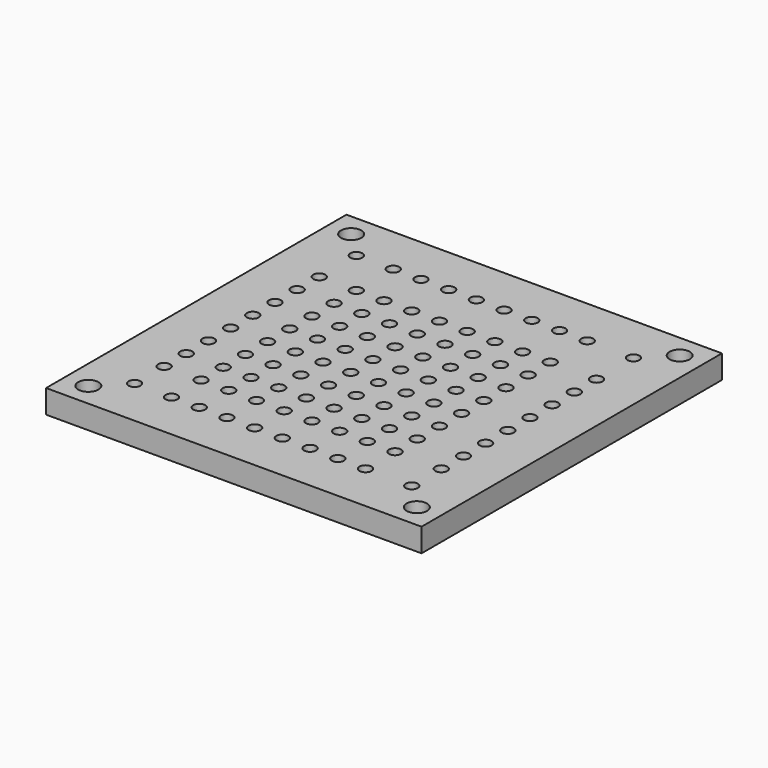
from build123d import *

# Parameters (mm, degrees)
F1_W     = 203.2
F1_H     = 203.2
F2_DEPTH = 12.7
F3_R     = 5.5
F3_R_2   = 3.25
F4_DEPTH = 6.35
F5_DEPTH = 12.701
F6_R     = 3.25
F7_DEPTH = 12.7
F8_DEPTH = 5


# Not quite as in the source:
# - a feature names something its author has since deleted; it is built from what else it names


with BuildPart() as f2:
    # F1 (on Top) → F2 (new body)
    with BuildSketch(Plane.XY):
        with Locations((101.6, 101.6)):
            Rectangle(F1_W, F1_H)
    extrude(amount=F2_DEPTH)

    # F3 (on face) → F4 (cut)
    with BuildSketch(Plane.XY.offset(12.7)):
        with Locations((12.7, 190.5)):
            Circle(F3_R)
        with Locations((12.7, 190.5)):
            Circle(F3_R_2, mode=Mode.SUBTRACT)
        with Locations((190.5, 190.5)):
            Circle(F3_R)
        with Locations((190.5, 190.5)):
            Circle(F3_R_2, mode=Mode.SUBTRACT)
        with Locations((190.5, 12.7)):
            Circle(F3_R)
        with Locations((190.5, 12.7)):
            Circle(F3_R_2, mode=Mode.SUBTRACT)
        with Locations((12.7, 12.7)):
            Circle(F3_R)
        with Locations((12.7, 12.7)):
            Circle(F3_R_2, mode=Mode.SUBTRACT)
        with Locations((12.7, 190.5)):
            Circle(F3_R_2)
        with Locations((190.5, 12.7)):
            Circle(F3_R_2)
        with Locations((190.5, 190.5)):
            Circle(F3_R_2)
        with Locations((12.7, 12.7)):
            Circle(F3_R_2)
    extrude(amount=-F4_DEPTH, mode=Mode.SUBTRACT)

    # F3 (on face) → F5 (cut, through all)
    with BuildSketch(Plane.XY.offset(12.7)):
        with Locations((12.7, 190.5)):
            Circle(F3_R_2)
        with Locations((190.5, 190.5)):
            Circle(F3_R_2)
        with Locations((190.5, 12.7)):
            Circle(F3_R_2)
        with Locations((12.7, 12.7)):
            Circle(F3_R_2)
    extrude(amount=-F5_DEPTH, mode=Mode.SUBTRACT)

    # F6 (on face) → F7 (cut, through all)
    with BuildSketch(Plane(origin=(0, 0, 0), x_dir=(1, 0, 0), z_dir=(0, 0, -1))):
        with Locations((26.6, -26.6)):
            Circle(F6_R)
        with Locations((46.6, -26.6)):
            Circle(F6_R)
        with Locations((61.6, -26.6)):
            Circle(F6_R)
        with Locations((76.6, -26.6)):
            Circle(F6_R)
        with Locations((91.6, -26.6)):
            Circle(F6_R)
        with Locations((106.6, -26.6)):
            Circle(F6_R)
        with Locations((121.6, -26.6)):
            Circle(F6_R)
        with Locations((136.6, -26.6)):
            Circle(F6_R)
        with Locations((151.6, -26.6)):
            Circle(F6_R)
        with Locations((176.6, -26.6)):
            Circle(F6_R)
        with Locations((176.6, -46.6)):
            Circle(F6_R)
        with Locations((151.6, -46.6)):
            Circle(F6_R)
        with Locations((136.6, -46.6)):
            Circle(F6_R)
        with Locations((121.6, -46.6)):
            Circle(F6_R)
        with Locations((106.6, -46.6)):
            Circle(F6_R)
        with Locations((91.6, -46.6)):
            Circle(F6_R)
        with Locations((76.6, -46.6)):
            Circle(F6_R)
        with Locations((61.6, -46.6)):
            Circle(F6_R)
        with Locations((46.6, -46.6)):
            Circle(F6_R)
        with Locations((26.6, -46.6)):
            Circle(F6_R)
        with Locations((26.6, -61.6)):
            Circle(F6_R)
        with Locations((46.6, -61.6)):
            Circle(F6_R)
        with Locations((61.6, -61.6)):
            Circle(F6_R)
        with Locations((76.6, -61.6)):
            Circle(F6_R)
        with Locations((91.6, -61.6)):
            Circle(F6_R)
        with Locations((106.6, -61.6)):
            Circle(F6_R)
        with Locations((121.6, -61.6)):
            Circle(F6_R)
        with Locations((136.6, -61.6)):
            Circle(F6_R)
        with Locations((151.6, -61.6)):
            Circle(F6_R)
        with Locations((176.6, -61.6)):
            Circle(F6_R)
        with Locations((176.6, -76.6)):
            Circle(F6_R)
        with Locations((151.6, -76.6)):
            Circle(F6_R)
        with Locations((136.6, -76.6)):
            Circle(F6_R)
        with Locations((121.6, -76.6)):
            Circle(F6_R)
        with Locations((106.6, -76.6)):
            Circle(F6_R)
        with Locations((91.6, -76.6)):
            Circle(F6_R)
        with Locations((76.6, -76.6)):
            Circle(F6_R)
        with Locations((61.6, -76.6)):
            Circle(F6_R)
        with Locations((46.6, -76.6)):
            Circle(F6_R)
        with Locations((26.6, -76.6)):
            Circle(F6_R)
        with Locations((26.6, -91.6)):
            Circle(F6_R)
        with Locations((46.6, -91.6)):
            Circle(F6_R)
        with Locations((61.6, -91.6)):
            Circle(F6_R)
        with Locations((76.6, -91.6)):
            Circle(F6_R)
        with Locations((91.6, -91.6)):
            Circle(F6_R)
        with Locations((106.6, -91.6)):
            Circle(F6_R)
        with Locations((121.6, -91.6)):
            Circle(F6_R)
        with Locations((136.6, -91.6)):
            Circle(F6_R)
        with Locations((151.6, -91.6)):
            Circle(F6_R)
        with Locations((176.6, -91.6)):
            Circle(F6_R)
        with Locations((176.6, -106.6)):
            Circle(F6_R)
        with Locations((151.6, -106.6)):
            Circle(F6_R)
        with Locations((136.6, -106.6)):
            Circle(F6_R)
        with Locations((121.6, -106.6)):
            Circle(F6_R)
        with Locations((106.6, -106.6)):
            Circle(F6_R)
        with Locations((91.6, -106.6)):
            Circle(F6_R)
        with Locations((76.6, -106.6)):
            Circle(F6_R)
        with Locations((61.6, -106.6)):
            Circle(F6_R)
        with Locations((46.6, -106.6)):
            Circle(F6_R)
        with Locations((26.6, -106.6)):
            Circle(F6_R)
        with Locations((26.6, -121.6)):
            Circle(F6_R)
        with Locations((46.6, -121.6)):
            Circle(F6_R)
        with Locations((61.6, -121.6)):
            Circle(F6_R)
        with Locations((76.6, -121.6)):
            Circle(F6_R)
        with Locations((91.6, -121.6)):
            Circle(F6_R)
        with Locations((106.6, -121.6)):
            Circle(F6_R)
        with Locations((121.6, -121.6)):
            Circle(F6_R)
        with Locations((136.6, -121.6)):
            Circle(F6_R)
        with Locations((151.6, -121.6)):
            Circle(F6_R)
        with Locations((176.6, -121.6)):
            Circle(F6_R)
        with Locations((176.6, -136.6)):
            Circle(F6_R)
        with Locations((151.6, -136.6)):
            Circle(F6_R)
        with Locations((136.6, -136.6)):
            Circle(F6_R)
        with Locations((121.6, -136.6)):
            Circle(F6_R)
        with Locations((106.6, -136.6)):
            Circle(F6_R)
        with Locations((91.6, -136.6)):
            Circle(F6_R)
        with Locations((76.6, -136.6)):
            Circle(F6_R)
        with Locations((61.6, -136.6)):
            Circle(F6_R)
        with Locations((46.6, -136.6)):
            Circle(F6_R)
        with Locations((26.6, -136.6)):
            Circle(F6_R)
        with Locations((26.6, -151.6)):
            Circle(F6_R)
        with Locations((46.6, -151.6)):
            Circle(F6_R)
        with Locations((61.6, -151.6)):
            Circle(F6_R)
        with Locations((76.6, -151.6)):
            Circle(F6_R)
        with Locations((91.6, -151.6)):
            Circle(F6_R)
        with Locations((106.6, -151.6)):
            Circle(F6_R)
        with Locations((121.6, -151.6)):
            Circle(F6_R)
        with Locations((136.6, -151.6)):
            Circle(F6_R)
        with Locations((151.6, -151.6)):
            Circle(F6_R)
        with Locations((176.6, -151.6)):
            Circle(F6_R)
        with Locations((176.6, -176.6)):
            Circle(F6_R)
        with Locations((151.6, -176.6)):
            Circle(F6_R)
        with Locations((136.6, -176.6)):
            Circle(F6_R)
        with Locations((121.6, -176.6)):
            Circle(F6_R)
        with Locations((106.6, -176.6)):
            Circle(F6_R)
        with Locations((91.6, -176.6)):
            Circle(F6_R)
        with Locations((76.6, -176.6)):
            Circle(F6_R)
        with Locations((61.6, -176.6)):
            Circle(F6_R)
        with Locations((46.6, -176.6)):
            Circle(F6_R)
        with Locations((26.6, -176.6)):
            Circle(F6_R)
    extrude(amount=-F7_DEPTH, mode=Mode.SUBTRACT)

    # F6 (on face) → F8 (cut)
    with BuildSketch(Plane(origin=(0, 0, 0), x_dir=(1, 0, 0), z_dir=(0, 0, -1))):
        Polygon((30.8457822208, -22.3542177792), (25.0459358482, -20.8001536274), (20.8001536274, -25.0459358482), (22.3542177792, -30.8457822208), (28.1540641518, -32.3998463726), (32.3998463726, -28.1540641518), align=None)
        with Locations((26.6, -26.6)):
            Circle(F6_R, mode=Mode.SUBTRACT)
        Polygon((50.8457822208, -22.3542177792), (45.0459358482, -20.8001536274), (40.8001536274, -25.0459358482), (42.3542177792, -30.8457822208), (48.1540641518, -32.3998463726), (52.3998463726, -28.1540641518), align=None)
        with Locations((46.6, -26.6)):
            Circle(F6_R, mode=Mode.SUBTRACT)
        Polygon((65.8457822208, -22.3542177792), (60.0459358482, -20.8001536274), (55.8001536274, -25.0459358482), (57.3542177792, -30.8457822208), (63.1540641518, -32.3998463726), (67.3998463726, -28.1540641518), align=None)
        with Locations((61.6, -26.6)):
            Circle(F6_R, mode=Mode.SUBTRACT)
        Polygon((80.8457822208, -22.3542177792), (75.0459358482, -20.8001536274), (70.8001536274, -25.0459358482), (72.3542177792, -30.8457822208), (78.1540641518, -32.3998463726), (82.3998463726, -28.1540641518), align=None)
        with Locations((76.6, -26.6)):
            Circle(F6_R, mode=Mode.SUBTRACT)
        Polygon((95.8457822208, -22.3542177792), (90.0459358482, -20.8001536274), (85.8001536274, -25.0459358482), (87.3542177792, -30.8457822208), (93.1540641518, -32.3998463726), (97.3998463726, -28.1540641518), align=None)
        with Locations((91.6, -26.6)):
            Circle(F6_R, mode=Mode.SUBTRACT)
        Polygon((110.8457822208, -22.3542177792), (105.0459358482, -20.8001536274), (100.8001536274, -25.0459358482), (102.3542177792, -30.8457822208), (108.1540641518, -32.3998463726), (112.3998463726, -28.1540641518), align=None)
        with Locations((106.6, -26.6)):
            Circle(F6_R, mode=Mode.SUBTRACT)
        Polygon((125.8457822208, -22.3542177792), (120.0459358482, -20.8001536274), (115.8001536274, -25.0459358482), (117.3542177792, -30.8457822208), (123.1540641518, -32.3998463726), (127.3998463726, -28.1540641518), align=None)
        with Locations((121.6, -26.6)):
            Circle(F6_R, mode=Mode.SUBTRACT)
        Polygon((140.8457822208, -22.3542177792), (135.0459358482, -20.8001536274), (130.8001536274, -25.0459358482), (132.3542177792, -30.8457822208), (138.1540641518, -32.3998463726), (142.3998463726, -28.1540641518), align=None)
        with Locations((136.6, -26.6)):
            Circle(F6_R, mode=Mode.SUBTRACT)
        Polygon((155.8457822208, -22.3542177792), (150.0459358482, -20.8001536274), (145.8001536274, -25.0459358482), (147.3542177792, -30.8457822208), (153.1540641518, -32.3998463726), (157.3998463726, -28.1540641518), align=None)
        with Locations((151.6, -26.6)):
            Circle(F6_R, mode=Mode.SUBTRACT)
        Polygon((180.8457822208, -22.3542177792), (175.0459358482, -20.8001536274), (170.8001536274, -25.0459358482), (172.3542177792, -30.8457822208), (178.1540641518, -32.3998463726), (182.3998463726, -28.1540641518), align=None)
        with Locations((176.6, -26.6)):
            Circle(F6_R, mode=Mode.SUBTRACT)
        Polygon((30.8457822208, -42.3542177792), (25.0459358482, -40.8001536274), (20.8001536274, -45.0459358482), (22.3542177792, -50.8457822208), (28.1540641518, -52.3998463726), (32.3998463726, -48.1540641518), align=None)
        with Locations((26.6, -46.6)):
            Circle(F6_R, mode=Mode.SUBTRACT)
        Polygon((50.8457822208, -42.3542177792), (45.0459358482, -40.8001536274), (40.8001536274, -45.0459358482), (42.3542177792, -50.8457822208), (48.1540641518, -52.3998463726), (52.3998463726, -48.1540641518), align=None)
        with Locations((46.6, -46.6)):
            Circle(F6_R, mode=Mode.SUBTRACT)
        Polygon((65.8457822208, -42.3542177792), (60.0459358482, -40.8001536274), (55.8001536274, -45.0459358482), (57.3542177792, -50.8457822208), (63.1540641518, -52.3998463726), (67.3998463726, -48.1540641518), align=None)
        with Locations((61.6, -46.6)):
            Circle(F6_R, mode=Mode.SUBTRACT)
        Polygon((80.8457822208, -42.3542177792), (75.0459358482, -40.8001536274), (70.8001536274, -45.0459358482), (72.3542177792, -50.8457822208), (78.1540641518, -52.3998463726), (82.3998463726, -48.1540641518), align=None)
        with Locations((76.6, -46.6)):
            Circle(F6_R, mode=Mode.SUBTRACT)
        Polygon((95.8457822208, -42.3542177792), (90.0459358482, -40.8001536274), (85.8001536274, -45.0459358482), (87.3542177792, -50.8457822208), (93.1540641518, -52.3998463726), (97.3998463726, -48.1540641518), align=None)
        with Locations((91.6, -46.6)):
            Circle(F6_R, mode=Mode.SUBTRACT)
        Polygon((110.8457822208, -42.3542177792), (105.0459358482, -40.8001536274), (100.8001536274, -45.0459358482), (102.3542177792, -50.8457822208), (108.1540641518, -52.3998463726), (112.3998463726, -48.1540641518), align=None)
        with Locations((106.6, -46.6)):
            Circle(F6_R, mode=Mode.SUBTRACT)
        Polygon((125.8457822208, -42.3542177792), (120.0459358482, -40.8001536274), (115.8001536274, -45.0459358482), (117.3542177792, -50.8457822208), (123.1540641518, -52.3998463726), (127.3998463726, -48.1540641518), align=None)
        with Locations((121.6, -46.6)):
            Circle(F6_R, mode=Mode.SUBTRACT)
        Polygon((140.8457822208, -42.3542177792), (135.0459358482, -40.8001536274), (130.8001536274, -45.0459358482), (132.3542177792, -50.8457822208), (138.1540641518, -52.3998463726), (142.3998463726, -48.1540641518), align=None)
        with Locations((136.6, -46.6)):
            Circle(F6_R, mode=Mode.SUBTRACT)
        Polygon((155.8457822208, -42.3542177792), (150.0459358482, -40.8001536274), (145.8001536274, -45.0459358482), (147.3542177792, -50.8457822208), (153.1540641518, -52.3998463726), (157.3998463726, -48.1540641518), align=None)
        with Locations((151.6, -46.6)):
            Circle(F6_R, mode=Mode.SUBTRACT)
        Polygon((180.8457822208, -42.3542177792), (175.0459358482, -40.8001536274), (170.8001536274, -45.0459358482), (172.3542177792, -50.8457822208), (178.1540641518, -52.3998463726), (182.3998463726, -48.1540641518), align=None)
        with Locations((176.6, -46.6)):
            Circle(F6_R, mode=Mode.SUBTRACT)
        Polygon((30.8457822208, -57.3542177792), (25.0459358482, -55.8001536274), (20.8001536274, -60.0459358482), (22.3542177792, -65.8457822208), (28.1540641518, -67.3998463726), (32.3998463726, -63.1540641518), align=None)
        with Locations((26.6, -61.6)):
            Circle(F6_R, mode=Mode.SUBTRACT)
        Polygon((50.8457822208, -57.3542177792), (45.0459358482, -55.8001536274), (40.8001536274, -60.0459358482), (42.3542177792, -65.8457822208), (48.1540641518, -67.3998463726), (52.3998463726, -63.1540641518), align=None)
        with Locations((46.6, -61.6)):
            Circle(F6_R, mode=Mode.SUBTRACT)
        Polygon((65.8457822208, -57.3542177792), (60.0459358482, -55.8001536274), (55.8001536274, -60.0459358482), (57.3542177792, -65.8457822208), (63.1540641518, -67.3998463726), (67.3998463726, -63.1540641518), align=None)
        with Locations((61.6, -61.6)):
            Circle(F6_R, mode=Mode.SUBTRACT)
        Polygon((80.8457822208, -57.3542177792), (75.0459358482, -55.8001536274), (70.8001536274, -60.0459358482), (72.3542177792, -65.8457822208), (78.1540641518, -67.3998463726), (82.3998463726, -63.1540641518), align=None)
        with Locations((76.6, -61.6)):
            Circle(F6_R, mode=Mode.SUBTRACT)
        Polygon((95.8457822208, -57.3542177792), (90.0459358482, -55.8001536274), (85.8001536274, -60.0459358482), (87.3542177792, -65.8457822208), (93.1540641518, -67.3998463726), (97.3998463726, -63.1540641518), align=None)
        with Locations((91.6, -61.6)):
            Circle(F6_R, mode=Mode.SUBTRACT)
        Polygon((110.8457822208, -57.3542177792), (105.0459358482, -55.8001536274), (100.8001536274, -60.0459358482), (102.3542177792, -65.8457822208), (108.1540641518, -67.3998463726), (112.3998463726, -63.1540641518), align=None)
        with Locations((106.6, -61.6)):
            Circle(F6_R, mode=Mode.SUBTRACT)
        Polygon((125.8457822208, -57.3542177792), (120.0459358482, -55.8001536274), (115.8001536274, -60.0459358482), (117.3542177792, -65.8457822208), (123.1540641518, -67.3998463726), (127.3998463726, -63.1540641518), align=None)
        with Locations((121.6, -61.6)):
            Circle(F6_R, mode=Mode.SUBTRACT)
        Polygon((140.8457822208, -57.3542177792), (135.0459358482, -55.8001536274), (130.8001536274, -60.0459358482), (132.3542177792, -65.8457822208), (138.1540641518, -67.3998463726), (142.3998463726, -63.1540641518), align=None)
        with Locations((136.6, -61.6)):
            Circle(F6_R, mode=Mode.SUBTRACT)
        Polygon((155.8457822208, -57.3542177792), (150.0459358482, -55.8001536274), (145.8001536274, -60.0459358482), (147.3542177792, -65.8457822208), (153.1540641518, -67.3998463726), (157.3998463726, -63.1540641518), align=None)
        with Locations((151.6, -61.6)):
            Circle(F6_R, mode=Mode.SUBTRACT)
        Polygon((180.8457822208, -57.3542177792), (175.0459358482, -55.8001536274), (170.8001536274, -60.0459358482), (172.3542177792, -65.8457822208), (178.1540641518, -67.3998463726), (182.3998463726, -63.1540641518), align=None)
        with Locations((176.6, -61.6)):
            Circle(F6_R, mode=Mode.SUBTRACT)
        Polygon((30.8457822208, -72.3542177792), (25.0459358482, -70.8001536274), (20.8001536274, -75.0459358482), (22.3542177792, -80.8457822208), (28.1540641518, -82.3998463726), (32.3998463726, -78.1540641518), align=None)
        with Locations((26.6, -76.6)):
            Circle(F6_R, mode=Mode.SUBTRACT)
        Polygon((50.8457822208, -72.3542177792), (45.0459358482, -70.8001536274), (40.8001536274, -75.0459358482), (42.3542177792, -80.8457822208), (48.1540641518, -82.3998463726), (52.3998463726, -78.1540641518), align=None)
        with Locations((46.6, -76.6)):
            Circle(F6_R, mode=Mode.SUBTRACT)
        Polygon((65.8457822208, -72.3542177792), (60.0459358482, -70.8001536274), (55.8001536274, -75.0459358482), (57.3542177792, -80.8457822208), (63.1540641518, -82.3998463726), (67.3998463726, -78.1540641518), align=None)
        with Locations((61.6, -76.6)):
            Circle(F6_R, mode=Mode.SUBTRACT)
        Polygon((80.8457822208, -72.3542177792), (75.0459358482, -70.8001536274), (70.8001536274, -75.0459358482), (72.3542177792, -80.8457822208), (78.1540641518, -82.3998463726), (82.3998463726, -78.1540641518), align=None)
        with Locations((76.6, -76.6)):
            Circle(F6_R, mode=Mode.SUBTRACT)
        Polygon((95.8457822208, -72.3542177792), (90.0459358482, -70.8001536274), (85.8001536274, -75.0459358482), (87.3542177792, -80.8457822208), (93.1540641518, -82.3998463726), (97.3998463726, -78.1540641518), align=None)
        with Locations((91.6, -76.6)):
            Circle(F6_R, mode=Mode.SUBTRACT)
        Polygon((110.8457822208, -72.3542177792), (105.0459358482, -70.8001536274), (100.8001536274, -75.0459358482), (102.3542177792, -80.8457822208), (108.1540641518, -82.3998463726), (112.3998463726, -78.1540641518), align=None)
        with Locations((106.6, -76.6)):
            Circle(F6_R, mode=Mode.SUBTRACT)
        Polygon((125.8457822208, -72.3542177792), (120.0459358482, -70.8001536274), (115.8001536274, -75.0459358482), (117.3542177792, -80.8457822208), (123.1540641518, -82.3998463726), (127.3998463726, -78.1540641518), align=None)
        with Locations((121.6, -76.6)):
            Circle(F6_R, mode=Mode.SUBTRACT)
        Polygon((140.8457822208, -72.3542177792), (135.0459358482, -70.8001536274), (130.8001536274, -75.0459358482), (132.3542177792, -80.8457822208), (138.1540641518, -82.3998463726), (142.3998463726, -78.1540641518), align=None)
        with Locations((136.6, -76.6)):
            Circle(F6_R, mode=Mode.SUBTRACT)
        Polygon((155.8457822208, -72.3542177792), (150.0459358482, -70.8001536274), (145.8001536274, -75.0459358482), (147.3542177792, -80.8457822208), (153.1540641518, -82.3998463726), (157.3998463726, -78.1540641518), align=None)
        with Locations((151.6, -76.6)):
            Circle(F6_R, mode=Mode.SUBTRACT)
        Polygon((180.8457822208, -72.3542177792), (175.0459358482, -70.8001536274), (170.8001536274, -75.0459358482), (172.3542177792, -80.8457822208), (178.1540641518, -82.3998463726), (182.3998463726, -78.1540641518), align=None)
        with Locations((176.6, -76.6)):
            Circle(F6_R, mode=Mode.SUBTRACT)
        Polygon((30.8457822208, -87.3542177792), (25.0459358482, -85.8001536274), (20.8001536274, -90.0459358482), (22.3542177792, -95.8457822208), (28.1540641518, -97.3998463726), (32.3998463726, -93.1540641518), align=None)
        with Locations((26.6, -91.6)):
            Circle(F6_R, mode=Mode.SUBTRACT)
        Polygon((50.8457822208, -87.3542177792), (45.0459358482, -85.8001536274), (40.8001536274, -90.0459358482), (42.3542177792, -95.8457822208), (48.1540641518, -97.3998463726), (52.3998463726, -93.1540641518), align=None)
        with Locations((46.6, -91.6)):
            Circle(F6_R, mode=Mode.SUBTRACT)
        Polygon((65.8457822208, -87.3542177792), (60.0459358482, -85.8001536274), (55.8001536274, -90.0459358482), (57.3542177792, -95.8457822208), (63.1540641518, -97.3998463726), (67.3998463726, -93.1540641518), align=None)
        with Locations((61.6, -91.6)):
            Circle(F6_R, mode=Mode.SUBTRACT)
        Polygon((80.8457822208, -87.3542177792), (75.0459358482, -85.8001536274), (70.8001536274, -90.0459358482), (72.3542177792, -95.8457822208), (78.1540641518, -97.3998463726), (82.3998463726, -93.1540641518), align=None)
        with Locations((76.6, -91.6)):
            Circle(F6_R, mode=Mode.SUBTRACT)
        Polygon((95.8457822208, -87.3542177792), (90.0459358482, -85.8001536274), (85.8001536274, -90.0459358482), (87.3542177792, -95.8457822208), (93.1540641518, -97.3998463726), (97.3998463726, -93.1540641518), align=None)
        with Locations((91.6, -91.6)):
            Circle(F6_R, mode=Mode.SUBTRACT)
        Polygon((110.8457822208, -87.3542177792), (105.0459358482, -85.8001536274), (100.8001536274, -90.0459358482), (102.3542177792, -95.8457822208), (108.1540641518, -97.3998463726), (112.3998463726, -93.1540641518), align=None)
        with Locations((106.6, -91.6)):
            Circle(F6_R, mode=Mode.SUBTRACT)
        Polygon((125.8457822208, -87.3542177792), (120.0459358482, -85.8001536274), (115.8001536274, -90.0459358482), (117.3542177792, -95.8457822208), (123.1540641518, -97.3998463726), (127.3998463726, -93.1540641518), align=None)
        with Locations((121.6, -91.6)):
            Circle(F6_R, mode=Mode.SUBTRACT)
        Polygon((140.8457822208, -87.3542177792), (135.0459358482, -85.8001536274), (130.8001536274, -90.0459358482), (132.3542177792, -95.8457822208), (138.1540641518, -97.3998463726), (142.3998463726, -93.1540641518), align=None)
        with Locations((136.6, -91.6)):
            Circle(F6_R, mode=Mode.SUBTRACT)
        Polygon((155.8457822208, -87.3542177792), (150.0459358482, -85.8001536274), (145.8001536274, -90.0459358482), (147.3542177792, -95.8457822208), (153.1540641518, -97.3998463726), (157.3998463726, -93.1540641518), align=None)
        with Locations((151.6, -91.6)):
            Circle(F6_R, mode=Mode.SUBTRACT)
        Polygon((180.8457822208, -87.3542177792), (175.0459358482, -85.8001536274), (170.8001536274, -90.0459358482), (172.3542177792, -95.8457822208), (178.1540641518, -97.3998463726), (182.3998463726, -93.1540641518), align=None)
        with Locations((176.6, -91.6)):
            Circle(F6_R, mode=Mode.SUBTRACT)
        Polygon((30.8457822208, -102.3542177792), (25.0459358482, -100.8001536274), (20.8001536274, -105.0459358482), (22.3542177792, -110.8457822208), (28.1540641518, -112.3998463726), (32.3998463726, -108.1540641518), align=None)
        with Locations((26.6, -106.6)):
            Circle(F6_R, mode=Mode.SUBTRACT)
        Polygon((50.8457822208, -102.3542177792), (45.0459358482, -100.8001536274), (40.8001536274, -105.0459358482), (42.3542177792, -110.8457822208), (48.1540641518, -112.3998463726), (52.3998463726, -108.1540641518), align=None)
        with Locations((46.6, -106.6)):
            Circle(F6_R, mode=Mode.SUBTRACT)
        Polygon((65.8457822208, -102.3542177792), (60.0459358482, -100.8001536274), (55.8001536274, -105.0459358482), (57.3542177792, -110.8457822208), (63.1540641518, -112.3998463726), (67.3998463726, -108.1540641518), align=None)
        with Locations((61.6, -106.6)):
            Circle(F6_R, mode=Mode.SUBTRACT)
        Polygon((80.8457822208, -102.3542177792), (75.0459358482, -100.8001536274), (70.8001536274, -105.0459358482), (72.3542177792, -110.8457822208), (78.1540641518, -112.3998463726), (82.3998463726, -108.1540641518), align=None)
        with Locations((76.6, -106.6)):
            Circle(F6_R, mode=Mode.SUBTRACT)
        Polygon((95.8457822208, -102.3542177792), (90.0459358482, -100.8001536274), (85.8001536274, -105.0459358482), (87.3542177792, -110.8457822208), (93.1540641518, -112.3998463726), (97.3998463726, -108.1540641518), align=None)
        with Locations((91.6, -106.6)):
            Circle(F6_R, mode=Mode.SUBTRACT)
        Polygon((110.8457822208, -102.3542177792), (105.0459358482, -100.8001536274), (100.8001536274, -105.0459358482), (102.3542177792, -110.8457822208), (108.1540641518, -112.3998463726), (112.3998463726, -108.1540641518), align=None)
        with Locations((106.6, -106.6)):
            Circle(F6_R, mode=Mode.SUBTRACT)
        Polygon((125.8457822208, -102.3542177792), (120.0459358482, -100.8001536274), (115.8001536274, -105.0459358482), (117.3542177792, -110.8457822208), (123.1540641518, -112.3998463726), (127.3998463726, -108.1540641518), align=None)
        with Locations((121.6, -106.6)):
            Circle(F6_R, mode=Mode.SUBTRACT)
        Polygon((140.8457822208, -102.3542177792), (135.0459358482, -100.8001536274), (130.8001536274, -105.0459358482), (132.3542177792, -110.8457822208), (138.1540641518, -112.3998463726), (142.3998463726, -108.1540641518), align=None)
        with Locations((136.6, -106.6)):
            Circle(F6_R, mode=Mode.SUBTRACT)
        Polygon((155.8457822208, -102.3542177792), (150.0459358482, -100.8001536274), (145.8001536274, -105.0459358482), (147.3542177792, -110.8457822208), (153.1540641518, -112.3998463726), (157.3998463726, -108.1540641518), align=None)
        with Locations((151.6, -106.6)):
            Circle(F6_R, mode=Mode.SUBTRACT)
        Polygon((180.8457822208, -102.3542177792), (175.0459358482, -100.8001536274), (170.8001536274, -105.0459358482), (172.3542177792, -110.8457822208), (178.1540641518, -112.3998463726), (182.3998463726, -108.1540641518), align=None)
        with Locations((176.6, -106.6)):
            Circle(F6_R, mode=Mode.SUBTRACT)
        Polygon((30.8457822208, -117.3542177792), (25.0459358482, -115.8001536274), (20.8001536274, -120.0459358482), (22.3542177792, -125.8457822208), (28.1540641518, -127.3998463726), (32.3998463726, -123.1540641518), align=None)
        with Locations((26.6, -121.6)):
            Circle(F6_R, mode=Mode.SUBTRACT)
        Polygon((50.8457822208, -117.3542177792), (45.0459358482, -115.8001536274), (40.8001536274, -120.0459358482), (42.3542177792, -125.8457822208), (48.1540641518, -127.3998463726), (52.3998463726, -123.1540641518), align=None)
        with Locations((46.6, -121.6)):
            Circle(F6_R, mode=Mode.SUBTRACT)
        Polygon((65.8457822208, -117.3542177792), (60.0459358482, -115.8001536274), (55.8001536274, -120.0459358482), (57.3542177792, -125.8457822208), (63.1540641518, -127.3998463726), (67.3998463726, -123.1540641518), align=None)
        with Locations((61.6, -121.6)):
            Circle(F6_R, mode=Mode.SUBTRACT)
        Polygon((80.8457822208, -117.3542177792), (75.0459358482, -115.8001536274), (70.8001536274, -120.0459358482), (72.3542177792, -125.8457822208), (78.1540641518, -127.3998463726), (82.3998463726, -123.1540641518), align=None)
        with Locations((76.6, -121.6)):
            Circle(F6_R, mode=Mode.SUBTRACT)
        Polygon((95.8457822208, -117.3542177792), (90.0459358482, -115.8001536274), (85.8001536274, -120.0459358482), (87.3542177792, -125.8457822208), (93.1540641518, -127.3998463726), (97.3998463726, -123.1540641518), align=None)
        with Locations((91.6, -121.6)):
            Circle(F6_R, mode=Mode.SUBTRACT)
        Polygon((110.8457822208, -117.3542177792), (105.0459358482, -115.8001536274), (100.8001536274, -120.0459358482), (102.3542177792, -125.8457822208), (108.1540641518, -127.3998463726), (112.3998463726, -123.1540641518), align=None)
        with Locations((106.6, -121.6)):
            Circle(F6_R, mode=Mode.SUBTRACT)
        Polygon((125.8457822208, -117.3542177792), (120.0459358482, -115.8001536274), (115.8001536274, -120.0459358482), (117.3542177792, -125.8457822208), (123.1540641518, -127.3998463726), (127.3998463726, -123.1540641518), align=None)
        with Locations((121.6, -121.6)):
            Circle(F6_R, mode=Mode.SUBTRACT)
        Polygon((140.8457822208, -117.3542177792), (135.0459358482, -115.8001536274), (130.8001536274, -120.0459358482), (132.3542177792, -125.8457822208), (138.1540641518, -127.3998463726), (142.3998463726, -123.1540641518), align=None)
        with Locations((136.6, -121.6)):
            Circle(F6_R, mode=Mode.SUBTRACT)
        Polygon((155.8457822208, -117.3542177792), (150.0459358482, -115.8001536274), (145.8001536274, -120.0459358482), (147.3542177792, -125.8457822208), (153.1540641518, -127.3998463726), (157.3998463726, -123.1540641518), align=None)
        with Locations((151.6, -121.6)):
            Circle(F6_R, mode=Mode.SUBTRACT)
        Polygon((180.8457822208, -117.3542177792), (175.0459358482, -115.8001536274), (170.8001536274, -120.0459358482), (172.3542177792, -125.8457822208), (178.1540641518, -127.3998463726), (182.3998463726, -123.1540641518), align=None)
        with Locations((176.6, -121.6)):
            Circle(F6_R, mode=Mode.SUBTRACT)
        Polygon((30.8457822208, -132.3542177792), (25.0459358482, -130.8001536274), (20.8001536274, -135.0459358482), (22.3542177792, -140.8457822208), (28.1540641518, -142.3998463726), (32.3998463726, -138.1540641518), align=None)
        with Locations((26.6, -136.6)):
            Circle(F6_R, mode=Mode.SUBTRACT)
        Polygon((50.8457822208, -132.3542177792), (45.0459358482, -130.8001536274), (40.8001536274, -135.0459358482), (42.3542177792, -140.8457822208), (48.1540641518, -142.3998463726), (52.3998463726, -138.1540641518), align=None)
        with Locations((46.6, -136.6)):
            Circle(F6_R, mode=Mode.SUBTRACT)
        Polygon((65.8457822208, -132.3542177792), (60.0459358482, -130.8001536274), (55.8001536274, -135.0459358482), (57.3542177792, -140.8457822208), (63.1540641518, -142.3998463726), (67.3998463726, -138.1540641518), align=None)
        with Locations((61.6, -136.6)):
            Circle(F6_R, mode=Mode.SUBTRACT)
        Polygon((80.8457822208, -132.3542177792), (75.0459358482, -130.8001536274), (70.8001536274, -135.0459358482), (72.3542177792, -140.8457822208), (78.1540641518, -142.3998463726), (82.3998463726, -138.1540641518), align=None)
        with Locations((76.6, -136.6)):
            Circle(F6_R, mode=Mode.SUBTRACT)
        Polygon((95.8457822208, -132.3542177792), (90.0459358482, -130.8001536274), (85.8001536274, -135.0459358482), (87.3542177792, -140.8457822208), (93.1540641518, -142.3998463726), (97.3998463726, -138.1540641518), align=None)
        with Locations((91.6, -136.6)):
            Circle(F6_R, mode=Mode.SUBTRACT)
        Polygon((110.8457822208, -132.3542177792), (105.0459358482, -130.8001536274), (100.8001536274, -135.0459358482), (102.3542177792, -140.8457822208), (108.1540641518, -142.3998463726), (112.3998463726, -138.1540641518), align=None)
        with Locations((106.6, -136.6)):
            Circle(F6_R, mode=Mode.SUBTRACT)
        Polygon((125.8457822208, -132.3542177792), (120.0459358482, -130.8001536274), (115.8001536274, -135.0459358482), (117.3542177792, -140.8457822208), (123.1540641518, -142.3998463726), (127.3998463726, -138.1540641518), align=None)
        with Locations((121.6, -136.6)):
            Circle(F6_R, mode=Mode.SUBTRACT)
        Polygon((140.8457822208, -132.3542177792), (135.0459358482, -130.8001536274), (130.8001536274, -135.0459358482), (132.3542177792, -140.8457822208), (138.1540641518, -142.3998463726), (142.3998463726, -138.1540641518), align=None)
        with Locations((136.6, -136.6)):
            Circle(F6_R, mode=Mode.SUBTRACT)
        Polygon((155.8457822208, -132.3542177792), (150.0459358482, -130.8001536274), (145.8001536274, -135.0459358482), (147.3542177792, -140.8457822208), (153.1540641518, -142.3998463726), (157.3998463726, -138.1540641518), align=None)
        with Locations((151.6, -136.6)):
            Circle(F6_R, mode=Mode.SUBTRACT)
        Polygon((180.8457822208, -132.3542177792), (175.0459358482, -130.8001536274), (170.8001536274, -135.0459358482), (172.3542177792, -140.8457822208), (178.1540641518, -142.3998463726), (182.3998463726, -138.1540641518), align=None)
        with Locations((176.6, -136.6)):
            Circle(F6_R, mode=Mode.SUBTRACT)
        Polygon((30.8457822208, -147.3542177792), (25.0459358482, -145.8001536274), (20.8001536274, -150.0459358482), (22.3542177792, -155.8457822208), (28.1540641518, -157.3998463726), (32.3998463726, -153.1540641518), align=None)
        with Locations((26.6, -151.6)):
            Circle(F6_R, mode=Mode.SUBTRACT)
        Polygon((50.8457822208, -147.3542177792), (45.0459358482, -145.8001536274), (40.8001536274, -150.0459358482), (42.3542177792, -155.8457822208), (48.1540641518, -157.3998463726), (52.3998463726, -153.1540641518), align=None)
        with Locations((46.6, -151.6)):
            Circle(F6_R, mode=Mode.SUBTRACT)
        Polygon((65.8457822208, -147.3542177792), (60.0459358482, -145.8001536274), (55.8001536274, -150.0459358482), (57.3542177792, -155.8457822208), (63.1540641518, -157.3998463726), (67.3998463726, -153.1540641518), align=None)
        with Locations((61.6, -151.6)):
            Circle(F6_R, mode=Mode.SUBTRACT)
        Polygon((80.8457822208, -147.3542177792), (75.0459358482, -145.8001536274), (70.8001536274, -150.0459358482), (72.3542177792, -155.8457822208), (78.1540641518, -157.3998463726), (82.3998463726, -153.1540641518), align=None)
        with Locations((76.6, -151.6)):
            Circle(F6_R, mode=Mode.SUBTRACT)
        Polygon((95.8457822208, -147.3542177792), (90.0459358482, -145.8001536274), (85.8001536274, -150.0459358482), (87.3542177792, -155.8457822208), (93.1540641518, -157.3998463726), (97.3998463726, -153.1540641518), align=None)
        with Locations((91.6, -151.6)):
            Circle(F6_R, mode=Mode.SUBTRACT)
        Polygon((110.8457822208, -147.3542177792), (105.0459358482, -145.8001536274), (100.8001536274, -150.0459358482), (102.3542177792, -155.8457822208), (108.1540641518, -157.3998463726), (112.3998463726, -153.1540641518), align=None)
        with Locations((106.6, -151.6)):
            Circle(F6_R, mode=Mode.SUBTRACT)
        Polygon((125.8457822208, -147.3542177792), (120.0459358482, -145.8001536274), (115.8001536274, -150.0459358482), (117.3542177792, -155.8457822208), (123.1540641518, -157.3998463726), (127.3998463726, -153.1540641518), align=None)
        with Locations((121.6, -151.6)):
            Circle(F6_R, mode=Mode.SUBTRACT)
        Polygon((140.8457822208, -147.3542177792), (135.0459358482, -145.8001536274), (130.8001536274, -150.0459358482), (132.3542177792, -155.8457822208), (138.1540641518, -157.3998463726), (142.3998463726, -153.1540641518), align=None)
        with Locations((136.6, -151.6)):
            Circle(F6_R, mode=Mode.SUBTRACT)
        Polygon((155.8457822208, -147.3542177792), (150.0459358482, -145.8001536274), (145.8001536274, -150.0459358482), (147.3542177792, -155.8457822208), (153.1540641518, -157.3998463726), (157.3998463726, -153.1540641518), align=None)
        with Locations((151.6, -151.6)):
            Circle(F6_R, mode=Mode.SUBTRACT)
        Polygon((180.8457822208, -147.3542177792), (175.0459358482, -145.8001536274), (170.8001536274, -150.0459358482), (172.3542177792, -155.8457822208), (178.1540641518, -157.3998463726), (182.3998463726, -153.1540641518), align=None)
        with Locations((176.6, -151.6)):
            Circle(F6_R, mode=Mode.SUBTRACT)
        Polygon((30.8457822208, -172.3542177792), (25.0459358482, -170.8001536274), (20.8001536274, -175.0459358482), (22.3542177792, -180.8457822208), (28.1540641518, -182.3998463726), (32.3998463726, -178.1540641518), align=None)
        with Locations((26.6, -176.6)):
            Circle(F6_R, mode=Mode.SUBTRACT)
        Polygon((50.8457822208, -172.3542177792), (45.0459358482, -170.8001536274), (40.8001536274, -175.0459358482), (42.3542177792, -180.8457822208), (48.1540641518, -182.3998463726), (52.3998463726, -178.1540641518), align=None)
        with Locations((46.6, -176.6)):
            Circle(F6_R, mode=Mode.SUBTRACT)
        Polygon((65.8457822208, -172.3542177792), (60.0459358482, -170.8001536274), (55.8001536274, -175.0459358482), (57.3542177792, -180.8457822208), (63.1540641518, -182.3998463726), (67.3998463726, -178.1540641518), align=None)
        with Locations((61.6, -176.6)):
            Circle(F6_R, mode=Mode.SUBTRACT)
        Polygon((80.8457822208, -172.3542177792), (75.0459358482, -170.8001536274), (70.8001536274, -175.0459358482), (72.3542177792, -180.8457822208), (78.1540641518, -182.3998463726), (82.3998463726, -178.1540641518), align=None)
        with Locations((76.6, -176.6)):
            Circle(F6_R, mode=Mode.SUBTRACT)
        Polygon((95.8457822208, -172.3542177792), (90.0459358482, -170.8001536274), (85.8001536274, -175.0459358482), (87.3542177792, -180.8457822208), (93.1540641518, -182.3998463726), (97.3998463726, -178.1540641518), align=None)
        with Locations((91.6, -176.6)):
            Circle(F6_R, mode=Mode.SUBTRACT)
        Polygon((110.8457822208, -172.3542177792), (105.0459358482, -170.8001536274), (100.8001536274, -175.0459358482), (102.3542177792, -180.8457822208), (108.1540641518, -182.3998463726), (112.3998463726, -178.1540641518), align=None)
        with Locations((106.6, -176.6)):
            Circle(F6_R, mode=Mode.SUBTRACT)
        Polygon((125.8457822208, -172.3542177792), (120.0459358482, -170.8001536274), (115.8001536274, -175.0459358482), (117.3542177792, -180.8457822208), (123.1540641518, -182.3998463726), (127.3998463726, -178.1540641518), align=None)
        with Locations((121.6, -176.6)):
            Circle(F6_R, mode=Mode.SUBTRACT)
        Polygon((140.8457822208, -172.3542177792), (135.0459358482, -170.8001536274), (130.8001536274, -175.0459358482), (132.3542177792, -180.8457822208), (138.1540641518, -182.3998463726), (142.3998463726, -178.1540641518), align=None)
        with Locations((136.6, -176.6)):
            Circle(F6_R, mode=Mode.SUBTRACT)
        Polygon((155.8457822208, -172.3542177792), (150.0459358482, -170.8001536274), (145.8001536274, -175.0459358482), (147.3542177792, -180.8457822208), (153.1540641518, -182.3998463726), (157.3998463726, -178.1540641518), align=None)
        with Locations((151.6, -176.6)):
            Circle(F6_R, mode=Mode.SUBTRACT)
        Polygon((180.8457822208, -172.3542177792), (175.0459358482, -170.8001536274), (170.8001536274, -175.0459358482), (172.3542177792, -180.8457822208), (178.1540641518, -182.3998463726), (182.3998463726, -178.1540641518), align=None)
        with Locations((176.6, -176.6)):
            Circle(F6_R, mode=Mode.SUBTRACT)
    extrude(amount=-F8_DEPTH, mode=Mode.SUBTRACT)


solid = f2.part
